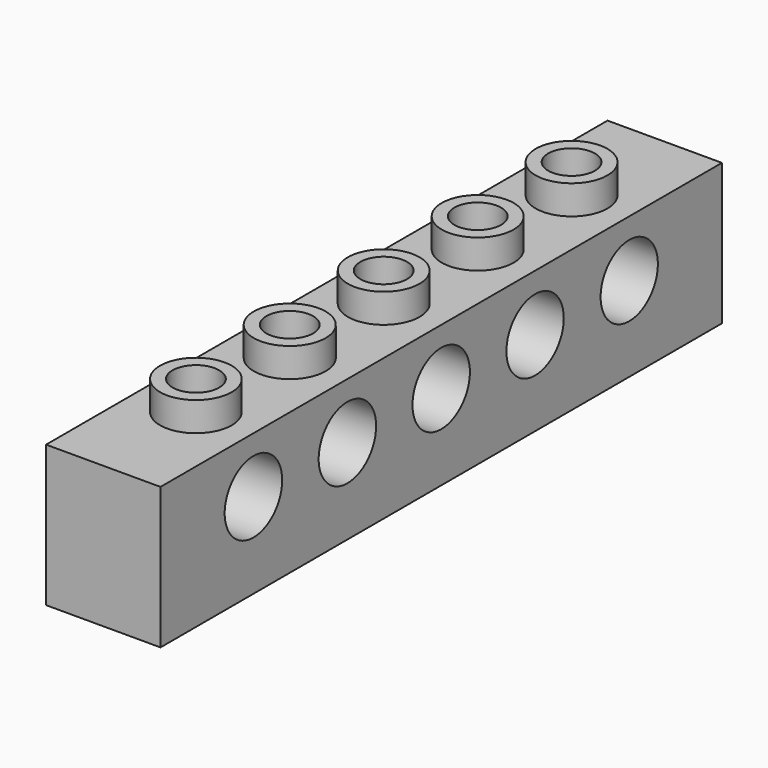
from build123d import *

# Parameters (mm, degrees)
F0_W      = 47.6758
F0_H      = 9.6012
F1_DEPTH  = 7.7724
F2_R      = 2.4384
F7_DEPTH  = 7.7724
F3_R      = 2.4352950492
F4_R      = 2.4324096057
F5_R      = 2.4384
F6_R      = 2.4411466666
F8_DEPTH  = 7.7724
F9_R      = 2.4401544128
F9_R_2    = 2.4440333998
F9_R_3    = 2.4447496076
F9_R_4    = 2.4340385208
F10_DEPTH = 1.9812
F11_R     = 2.4392424312
F12_DEPTH = 1.9812
F13_R     = 1.5875
F14_DEPTH = 1.9812
F15_T     = 1.4224
F16_R     = 1.5230861876
F16_R_2   = 1.5205363596
F16_R_3   = 1.5179209079
F16_R_4   = 1.5274772516
F16_R_5   = 1.526191219
F17_DEPTH = 1.9812


# Not quite as in the source:
# - a shell that OpenCascade refuses in one call is made with other operations: the cavity is built on its own and cut out


with BuildPart() as f1:
    # F0 (on Right) → F1 (new body)
    with BuildSketch(Plane.YZ):
        Rectangle(F0_W, F0_H)
    extrude(amount=F1_DEPTH)

    # F2 (on face) → F7 (cut, through all)
    with BuildSketch(Plane.YZ.offset(7.7724)):
        with Locations((0, 0.9964218903)):
            Circle(F2_R)
    extrude(amount=-F7_DEPTH, mode=Mode.SUBTRACT)

    # F3 (on face) + F4 (on face) + F5 (on face) + F6 (on face) → F8 (cut, through all)
    with BuildSketch(Plane.YZ.offset(7.7724)):
        with Locations((7.9721985385, 0.9674058529)):
            Circle(F3_R)
    with BuildSketch(Plane.YZ.offset(7.7724)):
        with Locations((15.967461552, 0.9593243012)):
            Circle(F4_R)
    with BuildSketch(Plane.YZ.offset(7.7724)):
        with Locations((-7.9666562378, 1.0009957477)):
            Circle(F5_R)
    with BuildSketch(Plane.YZ.offset(7.7724)):
        with Locations((-15.9450713545, 1.0028800461)):
            Circle(F6_R)
    extrude(amount=-F8_DEPTH, mode=Mode.SUBTRACT)

    # F9 (on face) → F10 (join)
    with BuildSketch(Plane.XY.offset(4.8006)):
        with Locations((3.8676063996, 15.9507207572)):
            Circle(F9_R)
        with Locations((3.8676063996, 7.9800710082)):
            Circle(F9_R_2)
        with Locations((3.8676063996, -7.9808151349)):
            Circle(F9_R_3)
        with Locations((3.8676063996, -15.9500315785)):
            Circle(F9_R_4)
    extrude(amount=F10_DEPTH)


with BuildPart() as f12:
    # F11 (on face) → F12 (new body)
    with BuildSketch(Plane.XY.offset(4.8006)):
        with Locations((3.8672508672, 0)):
            Circle(F11_R)
    extrude(amount=F12_DEPTH)


with BuildPart() as f14_tool:
    # F13 (on face) → F14 (new body, through all)
    with BuildSketch(Plane.XY.offset(4.8006)):
        with Locations((3.8676063996, -15.9500315785)):
            Circle(F13_R)
        with Locations((3.8676063996, -7.9808151349)):
            Circle(F13_R)
        with Locations((3.8672508672, 0)):
            Circle(F13_R)
        with Locations((3.8676063996, 7.9800710082)):
            Circle(F13_R)
        with Locations((3.8676063996, 15.9507207572)):
            Circle(F13_R)
    extrude(amount=F14_DEPTH)


with BuildPart() as f1_1:
    add(f1.part)

    # F14: cut by f14_tool
    add(f14_tool.part, mode=Mode.SUBTRACT)

    # F15: shell of thickness 1.4224, made by hand


with BuildPart() as f12_1:
    add(f12.part)

    # F14: cut by f14_tool
    add(f14_tool.part, mode=Mode.SUBTRACT)


with BuildPart() as f15_core1:
    # F15_t2: copy of F1
    add(f1_1.part)

    # the walls: a layer under each face that stays
    f15_faces = [f15_core1.faces().sort_by_distance(p)[0] for p in [
        (3.8862, -23.8379, 0),
        (3.8862, 23.8379, 0),
        (0, -15.8919333333, -3.2004),
        (7.7724, -15.8919333333, -3.2004),
        (3.8862, 0, 4.8006),
        (3.8862, 5.5369034893, 0.9674058529),
        (3.8862, 13.5350519463, 0.9593243012),
        (3.8862, -18.3862180211, 1.0028800461),
        (3.8862, -10.4050562378, 1.0009957477),
        (3.8862, -2.4384, 0.9964218903),
        (1.4274519868, 15.9507207572, 5.7912),
        (1.4235729997, 7.9800710082, 5.7912),
        (1.422856792, -7.9808151349, 5.7912),
        (1.4335678788, -15.9500315785, 5.7912),
        (2.2408367911, 14.3239511487, 6.7818),
        (2.2382507997, 6.3507154083, 6.7818),
        (2.2377733279, -9.6106482067, 6.7818),
        (2.2449140524, -17.5727239257, 6.7818),
        (2.2801063996, 15.9507207572, 5.7912),
        (2.2801063996, 7.9800710082, 5.7912),
        (2.2801063996, -7.9808151349, 5.7912),
        (2.2801063996, -15.9500315785, 5.7912),
        (3.8676063996, 15.9507207572, 4.8006),
        (3.8676063996, 7.9800710082, 4.8006),
        (3.8676063996, -7.9808151349, 4.8006),
        (3.8676063996, -15.9500315785, 4.8006),
    ]]
    thicken(f15_faces, amount=-F15_T, mode=Mode.SUBTRACT)

    # F15_s3 → F15_t4 (revolve, cut)
    with BuildSketch(Plane.XZ.offset(-15.9507207572)):
        Polygon((6.3219848124, 4.814824), (6.3077608124, 3.3782), (4.8853608124, 3.3782), (4.8853608124, 4.8006), align=None)
    revolve(axis=Axis((3.8676063996, 15.9507207572, 4.8006), (0, 0, 1)), mode=Mode.SUBTRACT)

    # F15_s5 → F15_t6 (revolve, cut)
    with BuildSketch(Plane.XZ.offset(-7.9800710082)):
        Polygon((6.3258637994, 4.814824), (6.3116397994, 3.3782), (4.8892397994, 3.3782), (4.8892397994, 4.8006), align=None)
    revolve(axis=Axis((3.8676063996, 7.9800710082, 4.8006), (0, 0, 1)), mode=Mode.SUBTRACT)

    # F15_s7 → F15_t8 (revolve, cut)
    with BuildSketch(Plane.XZ.offset(7.9808151349)):
        Polygon((6.3265800072, 4.814824), (6.3123560072, 3.3782), (4.8899560072, 3.3782), (4.8899560072, 4.8006), align=None)
    revolve(axis=Axis((3.8676063996, -7.9808151349, 4.8006), (0, 0, 1)), mode=Mode.SUBTRACT)

    # F15_s9 → F15_t10 (revolve, cut)
    with BuildSketch(Plane.XZ.offset(15.9500315785)):
        Polygon((6.3158689203, 4.814824), (6.3016449203, 3.3782), (4.8792449203, 3.3782), (4.8792449203, 4.8006), align=None)
    revolve(axis=Axis((3.8676063996, -15.9500315785, 4.8006), (0, 0, 1)), mode=Mode.SUBTRACT)

    # F15_s11 → F15_t12 (revolve, cut)
    with BuildSketch(Plane.XZ.offset(-15.9507207572)):
        Polygon((5.4408823996, 4.814824), (6.8775063996, 4.8006), (6.8775063996, 3.3782), (5.4551063996, 3.3782), align=None)
    revolve(axis=Axis((3.8676063996, 15.9507207572, 4.8006), (0, 0, 1)), mode=Mode.SUBTRACT)

    # F15_s13 → F15_t14 (revolve, cut)
    with BuildSketch(Plane.XZ.offset(-7.9800710082)):
        Polygon((5.4408823996, 4.814824), (6.8775063996, 4.8006), (6.8775063996, 3.3782), (5.4551063996, 3.3782), align=None)
    revolve(axis=Axis((3.8676063996, 7.9800710082, 4.8006), (0, 0, 1)), mode=Mode.SUBTRACT)

    # F15_s15 → F15_t16 (revolve, cut)
    with BuildSketch(Plane.XZ.offset(7.9808151349)):
        Polygon((5.4408823996, 4.814824), (6.8775063996, 4.8006), (6.8775063996, 3.3782), (5.4551063996, 3.3782), align=None)
    revolve(axis=Axis((3.8676063996, -7.9808151349, 4.8006), (0, 0, 1)), mode=Mode.SUBTRACT)

    # F15_s17 → F15_t18 (revolve, cut)
    with BuildSketch(Plane.XZ.offset(15.9500315785)):
        Polygon((5.4408823996, 4.814824), (6.8775063996, 4.8006), (6.8775063996, 3.3782), (5.4551063996, 3.3782), align=None)
    revolve(axis=Axis((3.8676063996, -15.9500315785, 4.8006), (0, 0, 1)), mode=Mode.SUBTRACT)


with BuildPart() as f1_2:
    add(f1_1.part)

    # what is left inside the walls is the cavity
    f15_cavity = [f15_core1.part.solids().sort_by_distance(p)[0] for p in [
        (4.707467, 0, -4.786376),
    ]]
    add(f15_cavity, mode=Mode.SUBTRACT)

    # F16 (on face) → F17 (join)
    with BuildSketch(Plane(origin=(0, 0, -4.8006), x_dir=(1, 0, 0), z_dir=(0, 0, -1))):
        with Locations((3.8792756386, -15.9459225833)):
            Circle(F16_R)
        with Locations((3.8792756386, -7.9726940021)):
            Circle(F16_R_2)
        with Locations((3.8792756386, 0)):
            Circle(F16_R_3)
        with Locations((3.8792756386, 7.9797049984)):
            Circle(F16_R_4)
        with Locations((3.8792756386, 15.9514807165)):
            Circle(F16_R_5)
    extrude(amount=-F17_DEPTH)


solid = Compound([f12_1.part, f1_2.part])
